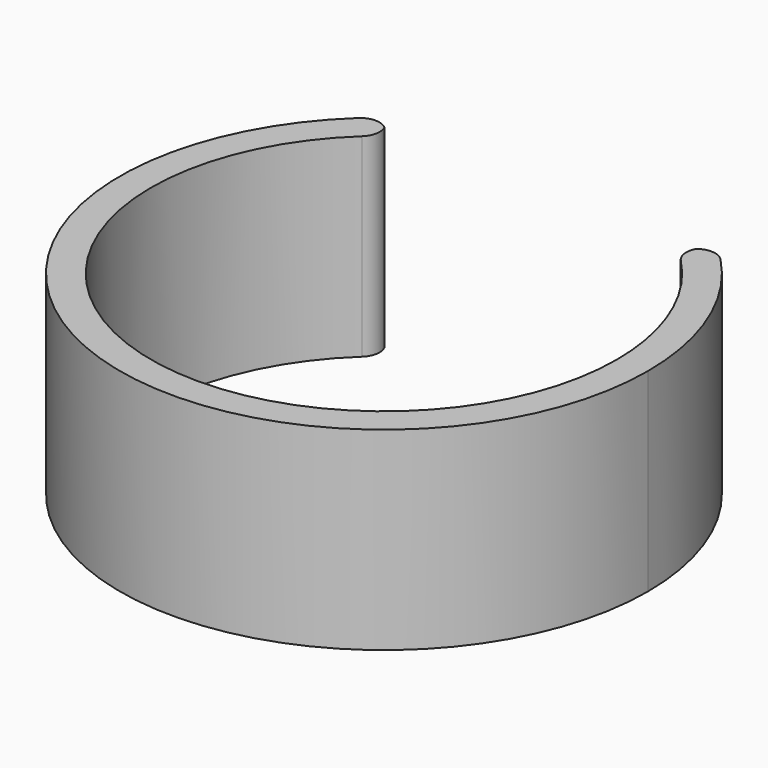
from build123d import *

# Parameters (mm, degrees)
F1_DEPTH    = 20
F2_T1_DEPTH = 29.6148139682
F2_T3_DEPTH = 30.8021727026


# Not quite as in the source:
# - a fillet or chamfer that OpenCascade refuses, or shapes differently, is made with other operations: its cross-section is extruded or revolved along the edge and cut away or added


with BuildPart() as f1:
    # F0 (on Top) → F1 (new body)
    with BuildSketch(Plane.XY):
        with BuildLine():
            ThreePointArc((15.9085457216, 17.9699241241), (21.8838421823, 9.8538039021), (24, 0))
            ThreePointArc((24, 0), (-10.4300926413, -21.6151143299), (-14.9344306245, 18.7873037427))
            Line((-14.9344306245, 18.7873037427), (-16.9256880412, 21.2922775751))
            ThreePointArc((-16.9256880411, 21.2922775751), (-11.8207716601, -24.4971295739), (27.2, 0))
            ThreePointArc((27.2, 0), (24.8016878066, 11.1676444224), (18.0296851511, 20.3659140073))
            Line((18.0296851511, 20.3659140073), (15.9085457216, 17.9699241241))
        make_face()
    extrude(amount=F1_DEPTH)

    # F2: fillet of radius 2 on 4 edges, made by hand

    # F2_s2 → F2_t1 (cut)
    with BuildSketch(Plane.XY.offset(-4.8074069841)):
        with BuildLine():
            ThreePointArc((-16.3353575734, 17.5828351795), (-15.7022990684, 18.8976894845), (-16.131028726, 20.2926073298))
            Line((-16.131028726, 20.2926073298), (-14.9344306245, 18.7873037427))
            ThreePointArc((-14.9344306245, 18.7873037427), (-15.6464884117, 18.1985548982), (-16.3353575734, 17.5828351795))
        make_face()
        with BuildLine():
            ThreePointArc((17.2437110419, 16.6929455011), (16.6811829734, 18.0394844298), (17.183193285, 19.4097364364))
            Line((17.183193285, 19.4097364364), (15.9085457216, 17.9699241241))
            ThreePointArc((15.9085457216, 17.9699241241), (16.5884206822, 17.3442872229), (17.2437110419, 16.6929455011))
        make_face()
    extrude(amount=F2_T1_DEPTH, mode=Mode.SUBTRACT)

    # F2_s4 → F2_t3 (cut)
    with BuildSketch(Plane.XY.offset(-5.4010863513)):
        with BuildLine():
            ThreePointArc((-18.5621612385, 19.8818050024), (-17.0493571531, 20.4144285626), (-15.6316877963, 19.6644434612))
            Line((-15.6316877963, 19.6644434612), (-16.9256880412, 21.2922775751))
            ThreePointArc((-16.9256880412, 21.2922775751), (-17.7579339971, 20.6032953713), (-18.5621612385, 19.8818050024))
        make_face()
        with BuildLine():
            ThreePointArc((19.5891550007, 18.8707447219), (18.1066850122, 19.482747002), (16.6512822795, 18.8089021064))
            Line((16.6512822795, 18.8089021064), (18.0296851511, 20.3659140073))
            ThreePointArc((18.0296851511, 20.3659140073), (18.8242706735, 19.6338186202), (19.5891550007, 18.8707447219))
        make_face()
    extrude(amount=F2_T3_DEPTH, mode=Mode.SUBTRACT)


solid = f1.part
